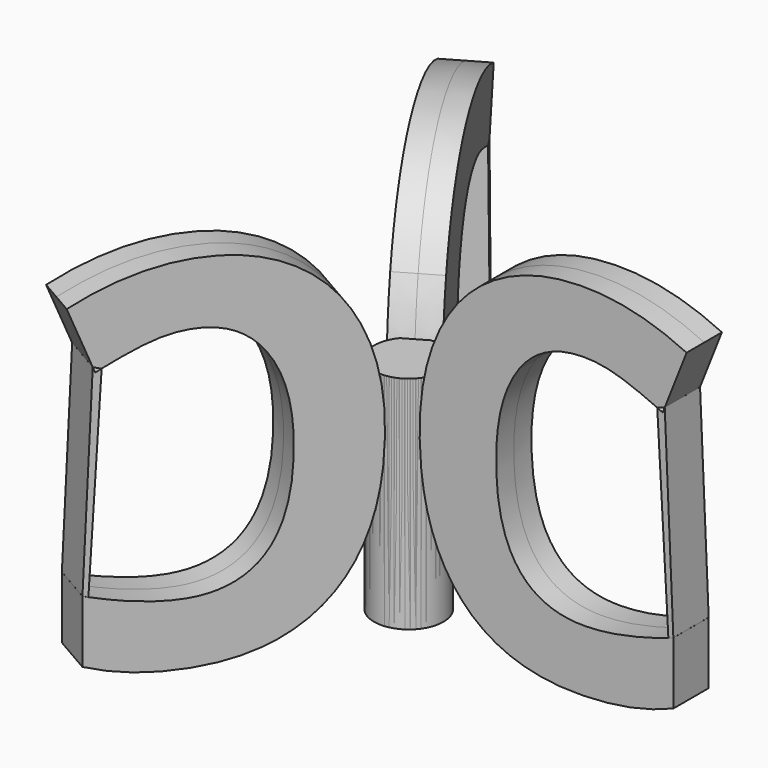
from build123d import *

# Parameters (mm, degrees)
F1_DEPTH = 2.5
F2_R     = 3.9262764501
F3_DEPTH = 25
F4_COUNT = 3
F5_COUNT = 3


# Not quite as in the source:
# - a feature names something its author has since deleted; it is built from what else it names


with BuildPart() as f1:
    # F0 (on Front) → F1 (new body, symmetric)
    with BuildSketch(Plane.XZ):
        with BuildLine():
            Line((30.14498758, 30.8754255745), (30.9688380118, 31.1823581479))
            Line((30.9688380118, 31.1823581479), (33.4461805556, 37.4392361111))
            add(Edge.make_bspline(
                [(21.8402777778, 40.2256944444), (27.6128472222, 40.2256944444), (33.4461805556, 37.4392361111)],
                knots=[0, 0, 0, 1, 1, 1], degree=2))
            add(Edge.make_bspline(
                [(11.953125, 37.7473958333), (16.171875, 40.2256944444), (21.8402777778, 40.2256944444)],
                knots=[0, 0, 0, 1, 1, 1], degree=2))
            add(Edge.make_bspline(
                [(5.4817708333, 30.6163194444), (7.734375, 35.2690972222), (11.953125, 37.7473958333)],
                knots=[0, 0, 0, 1, 1, 1], degree=2))
            add(Edge.make_bspline(
                [(3.2291666667, 19.7743055556), (3.2291666667, 25.9635416667), (5.4817708333, 30.6163194444)],
                knots=[0, 0, 0, 1, 1, 1], degree=2))
            add(Edge.make_bspline(
                [(7.8125, 4.7048611111), (3.2291666667, 9.9565972222), (3.2291666667, 19.7743055556)],
                knots=[0, 0, 0, 1, 1, 1], degree=2))
            add(Edge.make_bspline(
                [(21.0503472222, -0.546875), (12.3958333333, -0.546875), (7.8125, 4.7048611111)],
                knots=[0, 0, 0, 1, 1, 1], degree=2))
            add(Edge.make_bspline(
                [(31.953125, 1.4930555556), (27.0746527778, -0.546875), (21.0503472222, -0.546875)],
                knots=[0, 0, 0, 1, 1, 1], degree=2))
            Line((31.953125, 1.4930555556), (31.953125, 8.5416666667))
            add(Edge.make_bspline(
                [(31.8996877311, 8.5229464541), (31.9263885001, 8.5322854386), (31.953125, 8.5416666667)],
                knots=[0.9954970105, 0.9954970105, 0.9954970105, 1, 1, 1], degree=2))
            Line((31.8996877311, 8.5229464541), (31.3860476017, 8.3274208009))
            Line((31.3860476017, 8.3274208009), (31.385024739, 8.3457346861))
            add(Edge.make_bspline(
                [(21.8402777778, 6.4583333333), (25.8144377696, 6.4583333333), (31.385024739, 8.3457346861)],
                knots=[0, 0, 0, 0.9518154492, 0.9518154492, 0.9518154492], degree=2))
            add(Edge.make_bspline(
                [(11.8836805556, 19.7222222222), (11.8836805556, 6.4583333333), (21.8402777778, 6.4583333333)],
                knots=[0, 0, 0, 1, 1, 1], degree=2))
            add(Edge.make_bspline(
                [(14.4878472222, 29.6614583333), (11.8836805556, 26.09375), (11.8836805556, 19.7222222222)],
                knots=[0, 0, 0, 1, 1, 1], degree=2))
            add(Edge.make_bspline(
                [(21.8402777778, 33.2291666667), (17.0920138889, 33.2291666667), (14.4878472222, 29.6614583333)],
                knots=[0, 0, 0, 1, 1, 1], degree=2))
            add(Edge.make_bspline(
                [(26.2586805556, 32.4435763889), (24.0104166667, 33.2291666667), (21.8402777778, 33.2291666667)],
                knots=[0, 0, 0, 1, 1, 1], degree=2))
            add(Edge.make_bspline(
                [(30.14498758, 30.8754255745), (28.2083620701, 31.762317018), (26.2586805556, 32.4435763889)],
                knots=[0.1328057511, 0.1328057511, 0.1328057511, 1, 1, 1], degree=2))
        make_face()
    extrude(amount=F1_DEPTH, both=True)

    # F2 (on Top) → F3 (join)
    with BuildSketch(Plane.XY):
        Circle(F2_R)
    extrude(amount=F3_DEPTH)


with BuildPart() as f1b:
    # F0 (on Front) → F1, piece 2 (new body, symmetric)
    with BuildSketch(Plane.XZ):
        with BuildLine():
            Line((31.9473929703, 8.5411062464), (30.9723224491, 31.1836563051))
            Line((30.9723224491, 31.1836563051), (30.9688380118, 31.1823581479))
            Line((30.9688380118, 31.1823581479), (30.7378472222, 30.5989583333))
            add(Edge.make_bspline(
                [(30.7378472222, 30.5989583333), (30.4415705032, 30.7396033128), (30.14498758, 30.8754255745)],
                knots=[0, 0, 0, 0.1328057511, 0.1328057511, 0.1328057511], degree=2))
            Line((30.14498758, 30.8754255745), (30.1270745695, 30.8687519282))
            Line((30.1270745695, 30.8687519282), (31.385024739, 8.3457346861))
            add(Edge.make_bspline(
                [(31.385024739, 8.3457346861), (31.6406750719, 8.432352988), (31.8996877311, 8.5229464541)],
                knots=[0.9518154492, 0.9518154492, 0.9518154492, 0.9954970105, 0.9954970105, 0.9954970105], degree=2))
            Line((31.8996877311, 8.5229464541), (31.9473929703, 8.5411062464))
        make_face()
    extrude(amount=F1_DEPTH, both=True)


with BuildPart() as f4_1:
    # F4: instance of F1
    add(f1.part.rotate(Axis((0, 0, 0), (0, 0, -1)), 1 * 360 / F4_COUNT))


with BuildPart() as f4_2:
    # F4: instance of F1
    add(f1.part.rotate(Axis((0, 0, 0), (0, 0, -1)), 2 * 360 / F4_COUNT))


with BuildPart() as f5_1:
    # F5: instance of F1b
    add(f1b.part.rotate(Axis((0, 0, 0), (0, 0, -1)), 1 * 360 / F5_COUNT))


with BuildPart() as f5_2:
    # F5: instance of F1b
    add(f1b.part.rotate(Axis((0, 0, 0), (0, 0, -1)), 2 * 360 / F5_COUNT))


solid = Compound([f1.part, f1b.part, f4_1.part, f4_2.part, f5_1.part, f5_2.part])
